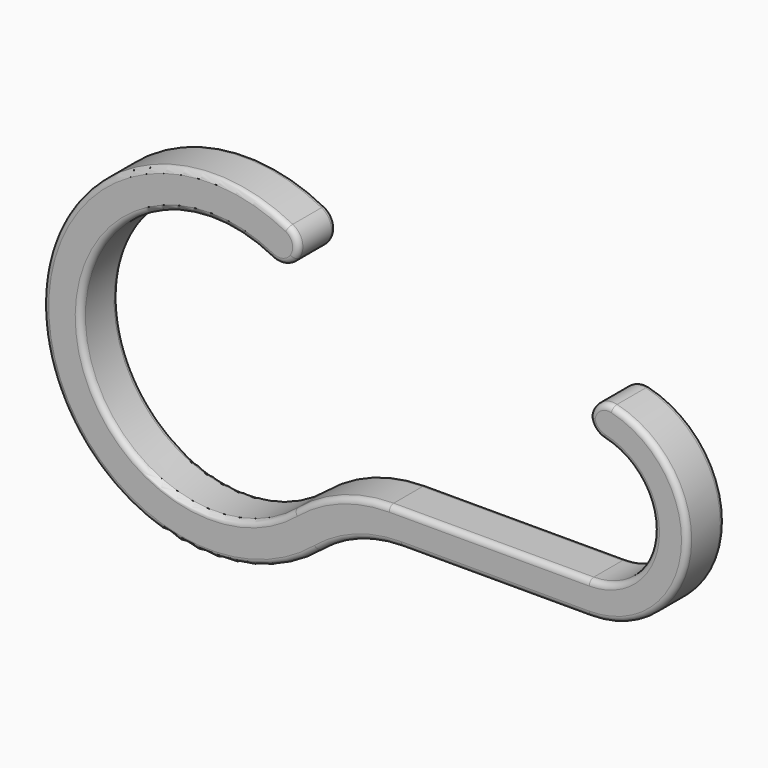
from build123d import *

# Parameters (mm, degrees)
F1_DEPTH     = 5
F2_T1_DEPTH  = 14.3624989998
F2_T3_DEPTH  = 16.2927187909
F2_T5_DEPTH  = 17.4769790167
F2_T7_DEPTH  = 13.8550247905
F3_T3_ANGLE  = 247.7046489152
F3_T6_ANGLE  = 113.0112311354
F3_T9_ANGLE  = 139.8913530699
F3_T12_ANGLE = 166.1930004756
F3_T15_DEPTH = 19.9331720401
F3_T18_ANGLE = 40
F3_T21_ANGLE = 247.7046489152
F3_T24_ANGLE = 97.2953510826
F3_T27_ANGLE = 82.7046489032
F3_T30_ANGLE = 247.704648915
F3_T33_ANGLE = 40
F3_T36_DEPTH = 21.2187472595
F3_T39_ANGLE = 166.9364387389
F3_T42_ANGLE = 97.2953510826
F3_T45_ANGLE = 40
F3_T48_DEPTH = 19.9331720401
F3_T51_ANGLE = 166.1930004756
F3_T54_ANGLE = 139.8913530699
F3_T57_ANGLE = 82.7046489032
F3_T60_ANGLE = 247.704648915
F3_T63_ANGLE = 40
F3_T66_DEPTH = 21.2187472595
F3_T69_ANGLE = 166.9364387389
F3_T72_ANGLE = 113.0112311354


# Not quite as in the source:
# - a fillet or chamfer that OpenCascade refuses, or shapes differently, is made with other operations: its cross-section is extruded or revolved along the edge and cut away or added


with BuildPart() as f1:
    # F0 (on Front) → F1 (new body)
    with BuildSketch(Plane.XZ):
        with BuildLine():
            ThreePointArc((8.8383296332, -10.5331110929), (-13.7369130468, -0.5997665763), (7.8866759998, 11.263340609))
            Line((7.8866759998, 11.263340609), (10.1809817452, 14.5399487861))
            ThreePointArc((10.1809817452, 14.5399487861), (-17.7331059331, -0.7742441257), (11.4094800719, -13.5972888654))
            ThreePointArc((11.4094800719, -13.5972888654), (15.5450327344, -11.2096264224), (20.2478097051, -10.3803999582))
            Line((20.2478097051, -10.3803999582), (40.1809817452, -10.3803999582))
            ThreePointArc((40.1809817452, -10.3803999582), (50.5613817035, 0), (40.1809817452, 10.3803999582))
            Line((40.1809817452, 10.3803999582), (40.1809817452, 6.848311072))
            ThreePointArc((40.1809817452, 6.848311072), (47.0292928172, 0), (40.1809817452, -6.848311072))
            Line((40.1809817452, -6.848311072), (18.9622344858, -6.848311072))
            ThreePointArc((18.9622344858, -6.848311072), (13.5754172284, -7.7981522946), (8.8383296332, -10.5331110929))
        make_face()
    extrude(amount=F1_DEPTH)

    # F2: fillet of radius 2 on 4 edges, made by hand

    # F2_s2 → F2_t1 (cut)
    with BuildSketch(Plane.XZ.offset(-4.6812494999)):
        with BuildLine():
            ThreePointArc((6.3925659055, 12.1736437086), (7.7942952649, 12.0008255138), (8.9606977622, 12.797202648))
            Line((8.9606977622, 12.797202648), (7.8866759998, 11.263340609))
            ThreePointArc((7.8866759998, 11.263340609), (7.1541142206, 11.7422804309), (6.3925659055, 12.1736437086))
        make_face()
    extrude(amount=F2_T1_DEPTH, mode=Mode.SUBTRACT)

    # F2_s4 → F2_t3 (cut)
    with BuildSketch(Plane.XZ.offset(-5.6463593955)):
        with BuildLine():
            ThreePointArc((8.9606977622, 12.797202648), (9.2659236806, 14.4162571121), (8.2522214417, 15.7150673329))
            ThreePointArc((8.2522214417, 15.7150673329), (9.2353110847, 15.1582165563), (10.1809817452, 14.5399487861))
            Line((10.1809817452, 14.5399487861), (8.9606977622, 12.797202648))
        make_face()
    extrude(amount=F2_T3_DEPTH, mode=Mode.SUBTRACT)

    # F2_s6 → F2_t5 (cut)
    with BuildSketch(Plane.XZ.offset(-6.2384895083)):
        with BuildLine():
            ThreePointArc((42.6582859336, 10.0804596746), (40.947006133, 9.7121948311), (40.1809817452, 8.1382494101))
            Line((40.1809817452, 8.1382494101), (40.1809817452, 10.3803999582))
            ThreePointArc((40.1809817452, 10.3803999582), (41.4286796469, 10.3051420776), (42.6582859336, 10.0804596746))
        make_face()
    extrude(amount=F2_T5_DEPTH, mode=Mode.SUBTRACT)

    # F2_s8 → F2_t7 (cut)
    with BuildSketch(Plane.XZ.offset(-4.4275123953)):
        with BuildLine():
            ThreePointArc((40.1809817452, 8.6193160301), (40.6150750837, 7.3751551372), (41.7289180726, 6.6710761999))
            ThreePointArc((41.7289180726, 6.6710761999), (40.9600066282, 6.8038580798), (40.1809817452, 6.848311072))
            Line((40.1809817452, 6.848311072), (40.1809817452, 8.6193160301))
        make_face()
    extrude(amount=F2_T7_DEPTH, mode=Mode.SUBTRACT)

    # F3: fillet of radius 0.6 on 13 edges, made by hand


with BuildPart() as f3_tool1:
    # F3_s2 → F3_t3 (revolve)
    with BuildSketch(Plane(origin=(0, 0, 0), x_dir=(0, 1, 0), z_dir=(0.8853559061, 0, -0.464913884))):
        with BuildLine():
            ThreePointArc((-5, 17.15), (-4.8242640687, 17.5742640687), (-4.4, 17.75))
            Line((-4.4, 17.75), (-5, 17.75))
            Line((-5, 17.75), (-5, 17.15))
        make_face()
    revolve(axis=Axis((0, -5, 0), (0, -1, 0)), revolution_arc=F3_T3_ANGLE)


with BuildPart() as f3_tool4:
    # F3_s5 → F3_t6 (revolve)
    with BuildSketch(Plane(origin=(38.1281196757, 0, -8.8471334716), x_dir=(0, 1, 0), z_dir=(0.9741199151, 0, -0.2260318363))):
        with BuildLine():
            ThreePointArc((0, 16.5304921614), (-0.1757359313, 16.1062280927), (-0.6, 15.9304921614))
            Line((-0.6, 15.9304921614), (0, 15.9304921614))
            Line((0, 15.9304921614), (0, 16.5304921614))
        make_face()
    revolve(axis=Axis((42.1809817453, 0, 8.6193160301), (0, 1, 0)), revolution_arc=F3_T6_ANGLE)


with BuildPart() as f3_tool7:
    # F3_s8 → F3_t9 (revolve)
    with BuildSketch(Plane(origin=(10.7586070612, 0, -14.762199147), x_dir=(0, 1, 0), z_dir=(0.5889756878, 0, -0.8081507528))):
        with BuildLine():
            ThreePointArc((0, 37.4818231941), (-0.1757359313, 37.0575591254), (-0.6, 36.8818231941))
            Line((-0.6, 36.8818231941), (0, 36.8818231941))
            Line((0, 36.8818231941), (0, 37.4818231941))
        make_face()
    revolve(axis=Axis((42.1809817452, 0, 8.13824941), (0, 1, 0)), revolution_arc=F3_T9_ANGLE)


with BuildPart() as f3_tool10:
    # F3_s11 → F3_t12 (revolve)
    with BuildSketch(Plane.YZ.offset(40.1809817452)):
        with BuildLine():
            ThreePointArc((0, -9.7803999582), (-0.1757359313, -10.204664027), (-0.6, -10.3803999582))
            Line((-0.6, -10.3803999582), (0, -10.3803999582))
            Line((0, -10.3803999582), (0, -9.7803999582))
        make_face()
    revolve(axis=Axis((40.1809817452, 0, 0), (0, -1, 0)), revolution_arc=F3_T12_ANGLE)


with BuildPart() as f3_tool13:
    # F3_s14 → F3_t15 (new body)
    with BuildSketch(Plane.YZ.offset(20.2478097051)):
        with BuildLine():
            ThreePointArc((0, -9.7803999582), (-0.1757359313, -10.204664027), (-0.6, -10.3803999582))
            Line((-0.6, -10.3803999582), (0, -10.3803999582))
            Line((0, -10.3803999582), (0, -9.7803999582))
        make_face()
    extrude(amount=F3_T15_DEPTH)


with BuildPart() as f3_tool16:
    # F3_s17 → F3_t18 (revolve)
    with BuildSketch(Plane(origin=(0, 0, 0), x_dir=(0, 1, 0), z_dir=(-0.7660444431, 0, -0.6427876097))):
        with BuildLine():
            ThreePointArc((0, 17.15), (-0.1757359313, 17.5742640687), (-0.6, 17.75))
            Line((-0.6, 17.75), (0, 17.75))
            Line((0, 17.75), (0, 17.15))
        make_face()
    revolve(axis=Axis((20.2478097051, 0, -24.1303999582), (0, 1, 0)), revolution_arc=F3_T18_ANGLE)


with BuildPart() as f3_tool19:
    # F3_s20 → F3_t21 (revolve)
    with BuildSketch(Plane(origin=(0, 0, 0), x_dir=(0, 1, 0), z_dir=(0.8853559061, 0, -0.464913884))):
        with BuildLine():
            ThreePointArc((0, 17.15), (-0.1757359313, 17.5742640687), (-0.6, 17.75))
            Line((-0.6, 17.75), (0, 17.75))
            Line((0, 17.75), (0, 17.15))
        make_face()
    revolve(axis=Axis((0, 0, 0), (0, -1, 0)), revolution_arc=F3_T21_ANGLE)


with BuildPart() as f3_tool22:
    # F3_s23 → F3_t24 (revolve)
    with BuildSketch(Plane(origin=(-3e-10, 0, 2e-10), x_dir=(0, 1, 0), z_dir=(-0.8853559061, 0, 0.4649138841))):
        with BuildLine():
            ThreePointArc((0, -17.15), (-0.1757359313, -17.5742640687), (-0.6, -17.75))
            Line((-0.6, -17.75), (0, -17.75))
            Line((0, -17.75), (0, -17.15))
        make_face()
    revolve(axis=Axis((7.3223936736, 0, 13.9443555207), (0, 1, 0)), revolution_arc=F3_T24_ANGLE)


with BuildPart() as f3_tool25:
    # F3_s26 → F3_t27 (revolve)
    with BuildSketch(Plane(origin=(8.9606977638, 0, 12.7972026469), x_dir=(0, 1, 0), z_dir=(0.5735764365, 0, 0.8191520442))):
        with BuildLine():
            ThreePointArc((0, 0.600000002), (-0.1757359313, 0.1757359332), (-0.6, 2e-09))
            Line((-0.6, 2e-09), (0, 2e-09))
            Line((0, 2e-09), (0, 0.600000002))
        make_face()
    revolve(axis=Axis((7.3223936736, 0, 13.9443555211), (0, 1, 0)), revolution_arc=F3_T27_ANGLE)


with BuildPart() as f3_tool28:
    # F3_s29 → F3_t30 (revolve)
    with BuildSketch(Plane(origin=(0, 0, 0), x_dir=(0, 1, 0), z_dir=(0.7660444431, 0, 0.6427876097))):
        with BuildLine():
            ThreePointArc((-0.6, -13.75), (-0.1757359313, -13.9257359313), (0, -14.35))
            Line((0, -14.35), (0, -13.75))
            Line((0, -13.75), (-0.6, -13.75))
        make_face()
    revolve(axis=Axis((0, 0, 0), (0, 1, 0)), revolution_arc=F3_T30_ANGLE)


with BuildPart() as f3_tool31:
    # F3_s32 → F3_t33 (revolve)
    with BuildSketch(Plane.YZ.offset(18.9622344858)):
        with BuildLine():
            ThreePointArc((0, -7.448311072), (-0.1757359313, -7.0240470033), (-0.6, -6.848311072))
            Line((-0.6, -6.848311072), (0, -6.848311072))
            Line((0, -6.848311072), (0, -7.448311072))
        make_face()
    revolve(axis=Axis((18.9622344858, 0, -22.598311072), (0, -1, 0)), revolution_arc=F3_T33_ANGLE)


with BuildPart() as f3_tool34:
    # F3_s35 → F3_t36 (new body)
    with BuildSketch(Plane.YZ.offset(40.1809817452)):
        with BuildLine():
            ThreePointArc((0, -7.448311072), (-0.1757359313, -7.0240470033), (-0.6, -6.848311072))
            Line((-0.6, -6.848311072), (0, -6.848311072))
            Line((0, -6.848311072), (0, -7.448311072))
        make_face()
    extrude(amount=-F3_T36_DEPTH)


with BuildPart() as f3_tool37:
    # F3_s38 → F3_t39 (revolve)
    with BuildSketch(Plane(origin=(38.1281196757, 0, -8.8471334717), x_dir=(0, 1, 0), z_dir=(-0.9741199151, 0, 0.2260318363))):
        with BuildLine():
            ThreePointArc((0, -16.5304921615), (-0.1757359313, -16.1062280928), (-0.6, -15.9304921615))
            Line((-0.6, -15.9304921615), (0, -15.9304921615))
            Line((0, -15.9304921615), (0, -16.5304921615))
        make_face()
    revolve(axis=Axis((40.1809817452, 0, 0), (0, 1, 0)), revolution_arc=F3_T39_ANGLE)


with BuildPart() as f3_tool40:
    # F3_s41 → F3_t42 (revolve)
    with BuildSketch(Plane(origin=(-3e-10, 0, 2e-10), x_dir=(0, 1, 0), z_dir=(-0.8853559061, 0, 0.4649138841))):
        with BuildLine():
            ThreePointArc((-5, -17.15), (-4.8242640687, -17.5742640687), (-4.4, -17.75))
            Line((-4.4, -17.75), (-5, -17.75))
            Line((-5, -17.75), (-5, -17.15))
        make_face()
    revolve(axis=Axis((7.3223936736, -5, 13.9443555207), (0, 1, 0)), revolution_arc=F3_T42_ANGLE)


with BuildPart() as f3_tool43:
    # F3_s44 → F3_t45 (revolve)
    with BuildSketch(Plane(origin=(0, 0, 0), x_dir=(0, 1, 0), z_dir=(-0.7660444431, 0, -0.6427876097))):
        with BuildLine():
            ThreePointArc((-5, 17.15), (-4.8242640687, 17.5742640687), (-4.4, 17.75))
            Line((-4.4, 17.75), (-5, 17.75))
            Line((-5, 17.75), (-5, 17.15))
        make_face()
    revolve(axis=Axis((20.2478097051, -5, -24.1303999582), (0, 1, 0)), revolution_arc=F3_T45_ANGLE)


with BuildPart() as f3_tool46:
    # F3_s47 → F3_t48 (new body)
    with BuildSketch(Plane.YZ.offset(20.2478097051)):
        with BuildLine():
            ThreePointArc((-5, -9.7803999582), (-4.8242640687, -10.204664027), (-4.4, -10.3803999582))
            Line((-4.4, -10.3803999582), (-5, -10.3803999582))
            Line((-5, -10.3803999582), (-5, -9.7803999582))
        make_face()
    extrude(amount=F3_T48_DEPTH)


with BuildPart() as f3_tool49:
    # F3_s50 → F3_t51 (revolve)
    with BuildSketch(Plane.YZ.offset(40.1809817452)):
        with BuildLine():
            ThreePointArc((-5, -9.7803999582), (-4.8242640687, -10.204664027), (-4.4, -10.3803999582))
            Line((-4.4, -10.3803999582), (-5, -10.3803999582))
            Line((-5, -10.3803999582), (-5, -9.7803999582))
        make_face()
    revolve(axis=Axis((40.1809817452, -5, 0), (0, -1, 0)), revolution_arc=F3_T51_ANGLE)


with BuildPart() as f3_tool52:
    # F3_s53 → F3_t54 (revolve)
    with BuildSketch(Plane(origin=(10.7586070612, 0, -14.762199147), x_dir=(0, 1, 0), z_dir=(0.5889756878, 0, -0.8081507528))):
        with BuildLine():
            ThreePointArc((-5, 37.4818231941), (-4.8242640687, 37.0575591254), (-4.4, 36.8818231941))
            Line((-4.4, 36.8818231941), (-5, 36.8818231941))
            Line((-5, 36.8818231941), (-5, 37.4818231941))
        make_face()
    revolve(axis=Axis((42.1809817452, -5, 8.13824941), (0, 1, 0)), revolution_arc=F3_T54_ANGLE)


with BuildPart() as f3_tool55:
    # F3_s56 → F3_t57 (revolve)
    with BuildSketch(Plane(origin=(8.9606977638, 0, 12.7972026469), x_dir=(0, 1, 0), z_dir=(0.5735764365, 0, 0.8191520442))):
        with BuildLine():
            ThreePointArc((-4.4, 2e-09), (-4.8242640687, 0.1757359332), (-5, 0.600000002))
            Line((-5, 0.600000002), (-5, 2e-09))
            Line((-5, 2e-09), (-4.4, 2e-09))
        make_face()
    revolve(axis=Axis((7.3223936736, -5, 13.9443555211), (0, 1, 0)), revolution_arc=F3_T57_ANGLE)


with BuildPart() as f3_tool58:
    # F3_s59 → F3_t60 (revolve)
    with BuildSketch(Plane(origin=(0, 0, 0), x_dir=(0, 1, 0), z_dir=(0.7660444431, 0, 0.6427876097))):
        with BuildLine():
            ThreePointArc((-4.4, -13.75), (-4.8242640687, -13.9257359313), (-5, -14.35))
            Line((-5, -14.35), (-5, -13.75))
            Line((-5, -13.75), (-4.4, -13.75))
        make_face()
    revolve(axis=Axis((0, -5, 0), (0, 1, 0)), revolution_arc=F3_T60_ANGLE)


with BuildPart() as f3_tool61:
    # F3_s62 → F3_t63 (revolve)
    with BuildSketch(Plane.YZ.offset(18.9622344858)):
        with BuildLine():
            ThreePointArc((-5, -7.448311072), (-4.8242640687, -7.0240470033), (-4.4, -6.848311072))
            Line((-4.4, -6.848311072), (-5, -6.848311072))
            Line((-5, -6.848311072), (-5, -7.448311072))
        make_face()
    revolve(axis=Axis((18.9622344858, -5, -22.598311072), (0, -1, 0)), revolution_arc=F3_T63_ANGLE)


with BuildPart() as f3_tool64:
    # F3_s65 → F3_t66 (new body)
    with BuildSketch(Plane.YZ.offset(40.1809817452)):
        with BuildLine():
            ThreePointArc((-5, -7.448311072), (-4.8242640687, -7.0240470033), (-4.4, -6.848311072))
            Line((-4.4, -6.848311072), (-5, -6.848311072))
            Line((-5, -6.848311072), (-5, -7.448311072))
        make_face()
    extrude(amount=-F3_T66_DEPTH)


with BuildPart() as f3_tool67:
    # F3_s68 → F3_t69 (revolve)
    with BuildSketch(Plane(origin=(38.1281196757, 0, -8.8471334717), x_dir=(0, 1, 0), z_dir=(-0.9741199151, 0, 0.2260318363))):
        with BuildLine():
            ThreePointArc((-5, -16.5304921615), (-4.8242640687, -16.1062280928), (-4.4, -15.9304921615))
            Line((-4.4, -15.9304921615), (-5, -15.9304921615))
            Line((-5, -15.9304921615), (-5, -16.5304921615))
        make_face()
    revolve(axis=Axis((40.1809817452, -5, 0), (0, 1, 0)), revolution_arc=F3_T69_ANGLE)


with BuildPart() as f3_tool70:
    # F3_s71 → F3_t72 (revolve)
    with BuildSketch(Plane(origin=(38.1281196757, 0, -8.8471334716), x_dir=(0, 1, 0), z_dir=(0.9741199151, 0, -0.2260318363))):
        with BuildLine():
            ThreePointArc((-5, 16.5304921614), (-4.8242640687, 16.1062280927), (-4.4, 15.9304921614))
            Line((-4.4, 15.9304921614), (-5, 15.9304921614))
            Line((-5, 15.9304921614), (-5, 16.5304921614))
        make_face()
    revolve(axis=Axis((42.1809817453, -5, 8.6193160301), (0, 1, 0)), revolution_arc=F3_T72_ANGLE)


with BuildPart() as f1_1:
    add(f1.part)

    # F3_t73: cut F3_tool1, F3_tool4, F3_tool7, F3_tool10, F3_tool13, F3_tool16, F3_tool19, F3_tool22, F3_tool25, F3_tool28, F3_tool31, F3_tool34, F3_tool37, F3_tool40, F3_tool43, F3_tool46, F3_tool49, F3_tool52, F3_tool55, F3_tool58, F3_tool61, F3_tool64, F3_tool67, F3_tool70
    add([f3_tool1.part, f3_tool4.part, f3_tool7.part, f3_tool10.part, f3_tool13.part, f3_tool16.part, f3_tool19.part, f3_tool22.part, f3_tool25.part, f3_tool28.part, f3_tool31.part, f3_tool34.part, f3_tool37.part, f3_tool40.part, f3_tool43.part, f3_tool46.part, f3_tool49.part, f3_tool52.part, f3_tool55.part, f3_tool58.part, f3_tool61.part, f3_tool64.part, f3_tool67.part, f3_tool70.part], mode=Mode.SUBTRACT)


solid = f1_1.part
